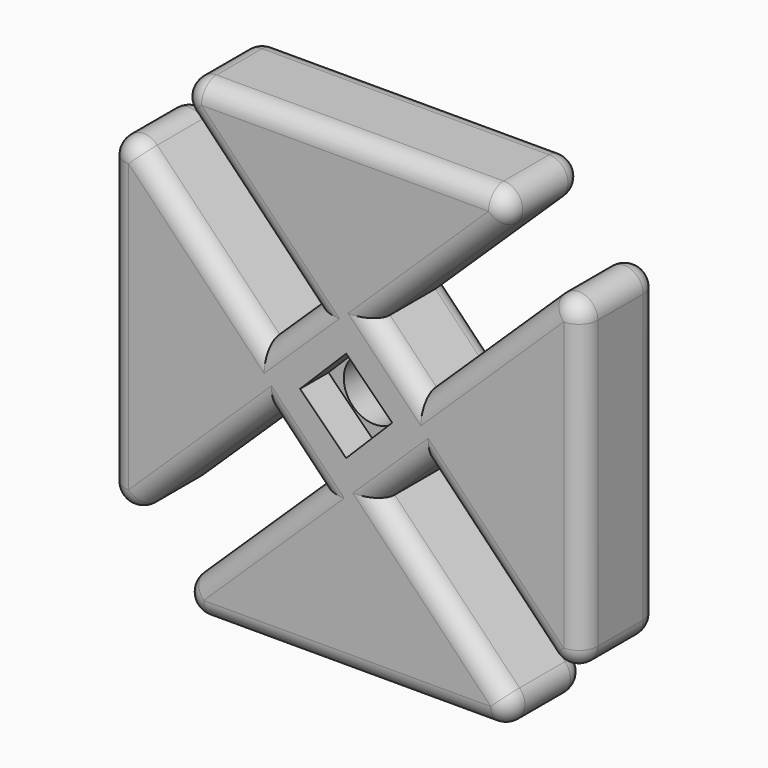
from build123d import *

# Parameters (mm, degrees)
F0_R     = 4.1148
F1_DEPTH = 12.7
F2_R     = 2.54
F5_DEPTH = 4.7498


# Not quite as in the source:
# - two fillets or chamfers of one size are made in one step
# - a feature of the source that left no trace in its solid (it failed there, or was rolled back) is left out
# - a feature names something its author has since deleted; it is built from what else it names


with BuildPart() as f1:
    # F0 (on Front) → F1 (new body)
    with BuildSketch(Plane.XZ):
        Polygon((27.9026240856, 20.8031311891), (6.35, 0), (57.15, 0), (36.2365272497, 21.6669410203), (42.6968688109, 27.9026240856), (63.5, 6.35), (63.5, 57.15), (41.8330589797, 36.2365272497), (35.5973759144, 42.6968688109), (57.15, 63.5), (6.35, 63.5), (27.2634727503, 41.8330589797), (20.8031311891, 35.5973759144), (0, 57.15), (0, 6.35), (21.6669410203, 27.2634727503), align=None)
        with Locations((31.75, 31.75)):
            Circle(F0_R, mode=Mode.SUBTRACT)
    extrude(amount=F1_DEPTH)

    # F2
    f2_edges = [f1.edges().sort_by_distance(p)[0] for p in [
        (31.75, -12.7, 63.5),
        (31.75, 0, 63.5),
        (10.401566, -12.7, 46.373688),
        (63.5, -12.7, 31.75),
        (31.75, -12.7, 0),
        (31.75, 0, 0),
        (0, -12.7, 31.75),
        (16.806736, -12.7, 52.666529),
        (24.033302, -12.7, 38.715217),
        (0, -6.35, 57.15),
        (6.35, -6.35, 63.5),
        (0, 0, 31.75),
        (24.784783, 0, 24.033302),
        (24.784783, -12.7, 24.033302),
        (6.35, -6.35, 0),
        (17.126312, 0, 10.401566),
        (17.126312, -12.7, 10.401566),
        (57.15, -6.35, 0),
        (46.693264, 0, 10.833471),
        (46.693264, -12.7, 10.833471),
        (39.466698, 0, 24.784783),
        (39.466698, -12.7, 24.784783),
        (63.5, -6.35, 6.35),
        (53.098434, 0, 17.126312),
        (53.098434, -12.7, 17.126312),
        (63.5, -6.35, 57.15),
        (63.5, 0, 31.75),
        (52.666529, 0, 46.693264),
        (52.666529, -12.7, 46.693264),
        (38.715217, 0, 39.466698),
        (38.715217, -12.7, 39.466698),
        (57.15, -6.35, 63.5),
        (46.373688, 0, 53.098434),
        (46.373688, -12.7, 53.098434),
        (16.806736, 0, 52.666529),
        (24.033302, 0, 38.715217),
        (10.401566, 0, 46.373688),
        (0, -6.35, 6.35),
        (10.833471, 0, 16.806736),
        (10.833471, -12.7, 16.806736),
    ]]
    fillet(f2_edges, radius=F2_R)

    # F4 (on face) → F5 (cut)
    with BuildSketch(Plane.XZ.offset(12.7)):
        Polygon((31.75, 25.5715837887), (37.9284162113, 31.75), (31.75, 37.9284162113), (25.5715837887, 31.75), align=None)
    extrude(amount=-F5_DEPTH, mode=Mode.SUBTRACT)


solid = f1.part
